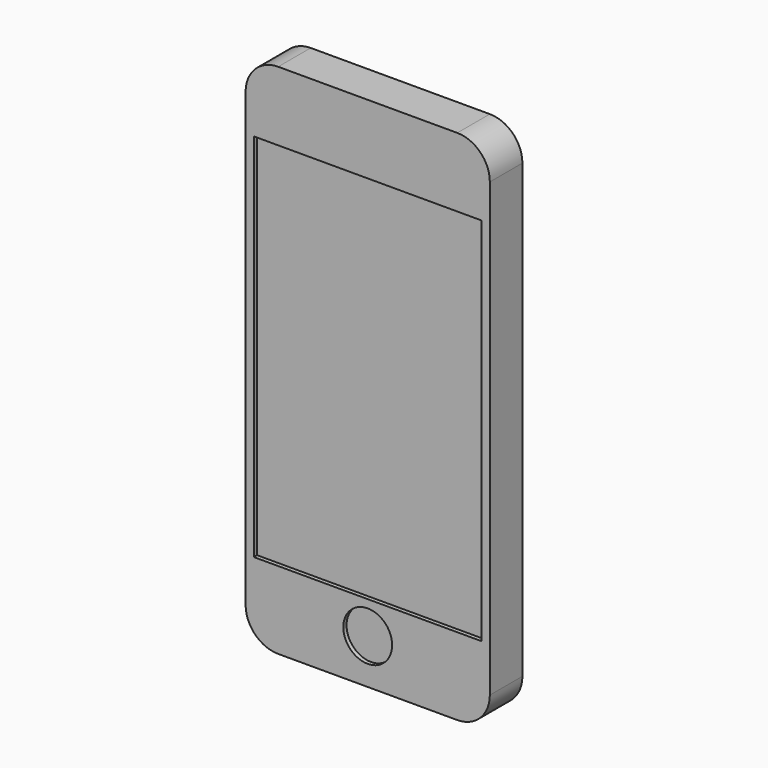
from build123d import *

# Parameters (mm, degrees)
F0_W     = 60
F0_H     = 127
F1_DEPTH = 10
F2_R     = 8
F3_R     = 6
F4_DEPTH = 1
F5_W     = 56
F5_H     = 91
F6_DEPTH = 1
F7_W     = 12
F7_H     = 4
F7_R     = 3
F8_DEPTH = 2
F9_R     = 1.99999
F10_R    = 0.5


# Not quite as in the source:
# - a fillet or chamfer is up to 0.001 mm smaller than in the source, because OpenCascade refuses the exact size


with BuildPart() as f1:
    # F0 (on Front) → F1 (new body)
    with BuildSketch(Plane.XZ):
        Rectangle(F0_W, F0_H)
    extrude(amount=F1_DEPTH)

    # F2
    f2_edges = [f1.edges().sort_by_distance(p)[0] for p in [
        (30, -5, 63.5),
        (-30, -5, 63.5),
        (30, -5, -63.5),
        (-30, -5, -63.5),
    ]]
    fillet(f2_edges, radius=F2_R)

    # F3 (on face) → F4 (cut)
    with BuildSketch(Plane.XZ.offset(10)):
        with Locations((0, -52.5)):
            Circle(F3_R)
    extrude(amount=-F4_DEPTH, mode=Mode.SUBTRACT)

    # F5 (on face) → F6 (cut)
    with BuildSketch(Plane.XZ.offset(10)):
        with Locations((0, 1)):
            Rectangle(F5_W, F5_H)
    extrude(amount=-F6_DEPTH, mode=Mode.SUBTRACT)

    # F7 (on face) → F8 (cut)
    with BuildSketch(Plane(origin=(0, 0, -63.5), x_dir=(1, 0, 0), z_dir=(0, 0, -1))):
        with Locations((0, 5)):
            Rectangle(F7_W, F7_H)
        with Locations((16, 5)):
            Rectangle(F7_W, F7_H)
        with Locations((-19, 5)):
            Circle(F7_R)
    extrude(amount=-F8_DEPTH, mode=Mode.SUBTRACT)

    # F9 (radius 2 in the source; OpenCascade refuses exactly that, so slightly less here)
    f9_edges = [f1.edges().sort_by_distance(p)[0] for p in [
        (-6, -7, -62.5),
        (-6, -3, -62.5),
        (6, -7, -62.5),
        (6, -3, -62.5),
    ]]
    fillet(f9_edges, radius=F9_R)

    # F10
    f10_edges = [f1.edges().sort_by_distance(p)[0] for p in [
        (10, -7, -62.5),
        (10, -3, -62.5),
        (22, -3, -62.5),
        (22, -7, -62.5),
    ]]
    fillet(f10_edges, radius=F10_R)


solid = f1.part
